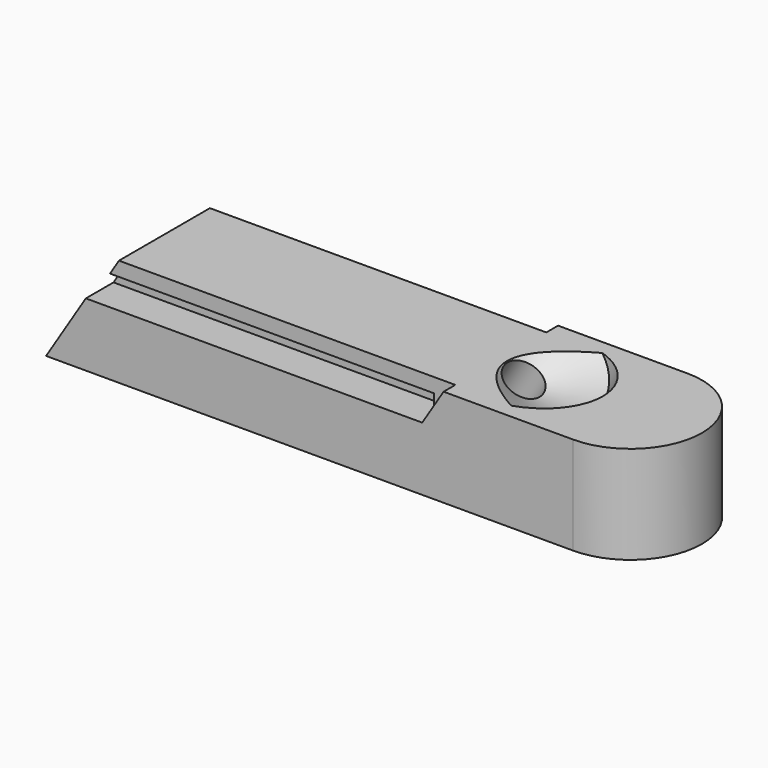
from build123d import *

# Parameters (mm, degrees)
F1_DEPTH = 6.2484
F3_DEPTH = 0.9398
F4_W     = 24.0350353877
F4_H     = 1.27
F5_DEPTH = 1.27
F7_DEPTH = 9.145


with BuildPart() as f1:
    # F0 (on Top) → F1 (new body)
    with BuildSketch(Plane.XY):
        with BuildLine():
            Line((10.287, 4.572), (-23.3934, 4.572))
            Line((-23.3934, 4.572), (-23.3934, -4.572))
            Line((-23.3934, -4.572), (10.287, -4.572))
            ThreePointArc((10.287, -4.572), (14.859, 0), (10.287, 4.572))
        make_face()
    extrude(amount=F1_DEPTH)

    # F2 (on face) → F3 (cut)
    with BuildSketch(Plane(origin=(0, 4.572, 0), x_dir=(-1, 0, 0), z_dir=(0, 1, 0))):
        Polygon((23.3934, 6.2484), (-2.0066, 6.2484), (-0.6416353877, 4.064), (23.3934, 4.064), align=None)
    extrude(amount=-F3_DEPTH, mode=Mode.SUBTRACT)

    # F4 (on face) → F5 (cut)
    with BuildSketch(Plane(origin=(0, 3.6322, 0), x_dir=(-1, 0, 0), z_dir=(0, 1, 0))):
        with Locations((11.3758823062, 4.699)):
            Rectangle(F4_W, F4_H)
    extrude(amount=-F5_DEPTH, mode=Mode.SUBTRACT)

    # F6 (on face) → F7 (cut, through all)
    with BuildSketch(Plane(origin=(0, 4.572, 0), x_dir=(-1, 0, 0), z_dir=(0, 1, 0))):
        Polygon((19.4889663415, 6.2484), (23.3934, 0), (23.3934, 6.2484), align=None)
    extrude(amount=-F7_DEPTH, mode=Mode.SUBTRACT)

    # F8: F1 across plane


with BuildPart() as f1_1:
    add(f1.part)
    add(f1.part.mirror(Plane.XZ), mode=Mode.INTERSECT)

    # F9 (on Front) → F10 (revolve, cut)
    with BuildSketch(Plane.XZ):
        Polygon((3.4612531172, 5.5391628772), (0, 0), (-1.3459949312, -2.1540421642), (-0.3228249031, -2.7933897565), (4.4844231452, 4.8998152849), align=None)
        Polygon((5.7204784574, 9.154679198), (3.4612531172, 5.5391628772), (4.4844231452, 4.8998152849), (7.6917084592, 4.9278048398), (9.0377033903, 7.081847004), align=None)
    revolve(axis=Axis((2.8602392287, 0, 4.577339599), (0.5299192642, 0, 0.8480480962)), mode=Mode.SUBTRACT)


solid = f1_1.part
